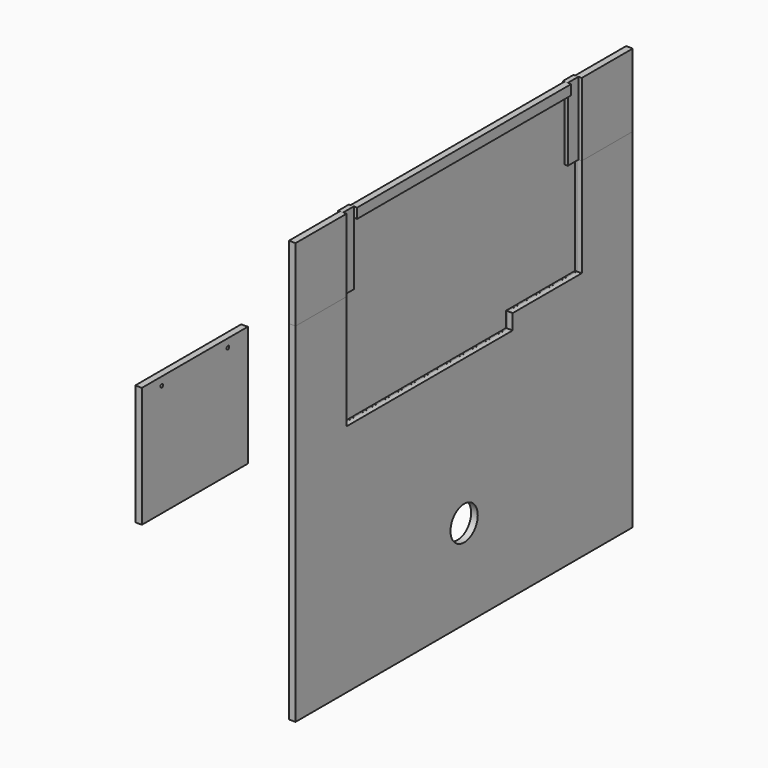
from build123d import *

# Parameters (mm, degrees)
F1_W          = 39.878
F1_H          = 36.322
F1_R          = 0.5
F2_DEPTH      = 2
F4_DEPTH      = 0.5
F5_T          = -0.01
F0_R          = 5.1320105677
F6_DEPTH      = 2
F0_R_2        = 0.005
F7_DEPTH      = 2
F0_W          = 4
F0_H          = 3
F0_H_2        = 19
F8_DEPTH      = 1
F8_DEPTH_BACK = 0.5


# Not quite as in the source:
# - the program builds the solid bodies; features that only make, move or delete a surface that nothing else refers to are left out


with BuildPart() as f2:
    # F1 (on Right) → F2 (new body)
    with BuildSketch(Plane.YZ):
        with Locations((-85.3744426475, 47.5188505783)):
            Rectangle(F1_W, F1_H)
        with Locations((-97.8306755424, 63.1798505783)):
            Circle(F1_R, mode=Mode.SUBTRACT)
        with Locations((-72.9284426475, 63.1798505783)):
            Circle(F1_R, mode=Mode.SUBTRACT)
    extrude(amount=F2_DEPTH)


with BuildPart() as f4:
    # F0 (on Right) → F4 (new body)
    with BuildSketch(Plane.YZ):
        Polygon((-24.2435368776, 58.5436199023), (-28.2435368776, 58.5436199023), (-28.2435368776, 24.1436199023), (34.3564631224, 24.1436199023), (34.3564631224, 28.7436199023), (34.3564631224, 77.5436199023), (-24.2435368776, 77.5436199023), align=None)
        Polygon((56.3564631224, 58.5436199023), (56.3564631224, 77.5436199023), (34.3564631224, 77.5436199023), (34.3564631224, 28.7436199023), (60.3564631224, 28.7436199023), (60.3564631224, 58.5436199023), align=None)
    extrude(amount=F4_DEPTH)

    # F5
    f5_openings = [f4.faces().sort_by_distance(p)[0] for p in [
        (0.5, 15.21705, 50.911751),
    ]]
    offset(amount=F5_T, openings=f5_openings, kind=Kind.INTERSECTION)


with BuildPart() as f6:
    # F0 (on Right) → F6 (new body)
    with BuildSketch(Plane.YZ):
        Polygon((-28.2435368776, 58.5436199023), (-47.4435368776, 58.5436199023), (-47.4435368776, -46.4563800977), (79.5564631224, -46.4563800977), (79.5564631224, 58.5436199023), (60.3564631224, 58.5436199023), (60.3564631224, 28.7436199023), (34.3564631224, 28.7436199023), (34.3564631224, 24.1436199023), (-28.2435368776, 24.1436199023), align=None)
        with Locations((16.0564631224, -19.5390637964)):
            Circle(F0_R, mode=Mode.SUBTRACT)
    extrude(amount=F6_DEPTH)


with BuildPart() as f7:
    # F0 (on Right) → F7 (new body)
    with BuildSketch(Plane.YZ):
        Polygon((-28.2435368776, 80.5436199023), (-47.4435368776, 80.5436199023), (-47.4435368776, 58.5436199023), (-28.2435368776, 58.5436199023), (-28.2435368776, 77.5436199023), align=None)
        with Locations((-38.3837649822, 80.4212242365)):
            Circle(F0_R_2, mode=Mode.SUBTRACT)
        with Locations((-37.3837649822, 80.4212242365)):
            Circle(F0_R_2, mode=Mode.SUBTRACT)
    extrude(amount=F7_DEPTH)


with BuildPart() as f7b:
    # F0 (on Right) → F7, piece 2 (new body)
    with BuildSketch(Plane.YZ):
        Polygon((79.5564631224, 80.5436199023), (60.3564631224, 80.5436199023), (60.3564631224, 77.5436199023), (60.3564631224, 58.5436199023), (79.5564631224, 58.5436199023), align=None)
        with Locations((69.4271420836, 80.4418772459)):
            Circle(F0_R_2, mode=Mode.SUBTRACT)
        with Locations((70.4271420836, 80.4418772459)):
            Circle(F0_R_2, mode=Mode.SUBTRACT)
    extrude(amount=F7_DEPTH)


with BuildPart() as f7c:
    # F0 (on Right) → F7, piece 3 (new body)
    with BuildSketch(Plane.YZ):
        Polygon((56.3564631224, 80.5436199023), (-24.2435368776, 80.5436199023), (-24.2435368776, 77.5436199023), (34.3564631224, 77.5436199023), (56.3564631224, 77.5436199023), align=None)
    extrude(amount=F7_DEPTH)


with BuildPart() as f8:
    # F0 (on Right) → F8 (new body, two sides)
    with BuildSketch(Plane.YZ) as f8_sk:
        with Locations((-26.2435368776, 79.0436199023)):
            Rectangle(F0_W, F0_H)
        with Locations((-26.2435368776, 68.0436199023)):
            Rectangle(F0_W, F0_H_2)
    extrude(amount=F8_DEPTH)
    extrude(f8_sk.sketch, amount=-F8_DEPTH_BACK)


with BuildPart() as f8b:
    # F0 (on Right) → F8, piece 2 (new body, two sides)
    with BuildSketch(Plane.YZ) as f8_2_sk:
        with Locations((58.3564631224, 79.0436199023)):
            Rectangle(F0_W, F0_H)
        with Locations((58.3564631224, 68.0436199023)):
            Rectangle(F0_W, F0_H_2)
    extrude(amount=F8_DEPTH)
    extrude(f8_2_sk.sketch, amount=-F8_DEPTH_BACK)


solid = Compound([f2.part, f4.part, f6.part, f7.part, f7b.part, f7c.part, f8.part, f8b.part])
